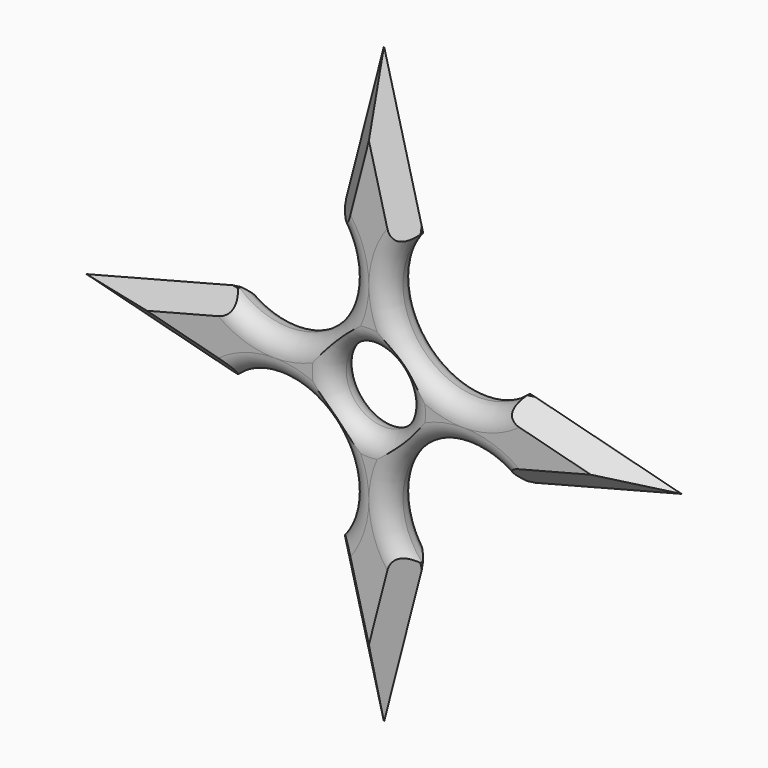
from build123d import *

# Parameters (mm, degrees)
F0_W         = 19.05
F0_H         = 25.4
F0_W_2       = 25.4
F0_H_2       = 19.05
F1_DEPTH     = 12.7
F3_D         = 50.8
F4_SIZE2     = 6.34999
F4_SIZE      = 6.34999
F5_T6_ANGLE  = 208.6059171241
F5_T8_ANGLE  = 208.6059171241
F5_T10_ANGLE = 208.6059171241
F5_T12_ANGLE = 208.6059171241
F5_T14_ANGLE = 208.6059171241
F5_T16_ANGLE = 208.6059171241
F5_T18_ANGLE = 208.6059171241
F5_T20_ANGLE = 208.6059171241


# Not quite as in the source:
# - a fillet or chamfer that OpenCascade refuses, or shapes differently, is made with other operations: its cross-section is extruded or revolved along the edge and cut away or added
# - a fillet or chamfer is up to 0.001 mm smaller than in the source, because OpenCascade refuses the exact size


with BuildPart() as f1:
    # F0 (on Front) → F1 (new body)
    with BuildSketch(Plane.XZ):
        with BuildLine():
            Line((-12.7, 12.7), (-4.87e-08, 12.7))
            Line((-4.87e-08, 12.7), (12.7, 12.7))
            Line((12.7, 12.7), (12.7, 14.1990316571))
            ThreePointArc((12.7, 14.1990316571), (0, 19.05), (-12.7, 14.1990316571))
            Line((-12.7, 14.1990316571), (-12.7, 12.7))
        make_face()
        with BuildLine():
            Line((-12.7, -12.7), (-12.7, 0))
            Line((-12.7, 0), (-12.7, 12.7))
            Line((-12.7, 12.7), (-14.1990316571, 12.7))
            ThreePointArc((-14.1990316571, 12.7), (-19.05, 0), (-14.1990316571, -12.7))
            Line((-14.1990316571, -12.7), (-12.7, -12.7))
        make_face()
        with BuildLine():
            Line((12.7, -12.7), (6e-10, -12.7))
            Line((6e-10, -12.7), (-12.7, -12.7))
            Line((-12.7, -12.7), (-12.7, -14.1990316571))
            ThreePointArc((-12.7, -14.1990316571), (0, -19.05), (12.7, -14.1990316571))
            Line((12.7, -14.1990316571), (12.7, -12.7))
        make_face()
        with BuildLine():
            Line((12.7, 12.7), (12.7, 0))
            Line((12.7, 0), (12.7, -12.7))
            Line((12.7, -12.7), (14.1990316571, -12.7))
            ThreePointArc((14.1990316571, -12.7), (17.7959834382, -6.7974608102), (19.05, 0))
            ThreePointArc((19.05, 0), (17.7959834382, 6.7974608102), (14.1990316571, 12.7))
            Line((14.1990316571, 12.7), (12.7, 12.7))
        make_face()
        with BuildLine():
            Line((12.7, -12.7), (12.7, 0))
            ThreePointArc((12.7, 0), (8.9802561213, -8.9802561208), (6e-10, -12.7))
            Line((6e-10, -12.7), (12.7, -12.7))
        make_face()
        with BuildLine():
            Line((-12.7, -12.7), (6e-10, -12.7))
            ThreePointArc((6e-10, -12.7), (-8.9802561208, -8.9802561213), (-12.7, 0))
            Line((-12.7, 0), (-12.7, -12.7))
        make_face()
        with BuildLine():
            ThreePointArc((-12.7, 0), (-8.9802561383, 8.9802561039), (-4.87e-08, 12.7))
            Line((-4.87e-08, 12.7), (-12.7, 12.7))
            Line((-12.7, 12.7), (-12.7, 0))
        make_face()
        with BuildLine():
            ThreePointArc((-4.87e-08, 12.7), (8.9802561039, 8.9802561383), (12.7, 0))
            Line((12.7, 0), (12.7, 12.7))
            Line((12.7, 12.7), (-4.87e-08, 12.7))
        make_face()
        with BuildLine():
            Line((12.7, 31.75), (12.7, 14.1990316571))
            ThreePointArc((12.7, 14.1990316571), (13.4703841816, 13.4703841816), (14.1990316571, 12.7))
            Line((14.1990316571, 12.7), (31.75, 12.7))
            Line((31.75, 12.7), (31.75, 31.75))
            Line((31.75, 31.75), (12.7, 31.75))
        make_face()
        with BuildLine():
            ThreePointArc((-12.7, 14.1990316571), (0, 19.05), (12.7, 14.1990316571))
            Line((12.7, 14.1990316571), (12.7, 31.75))
            Line((12.7, 31.75), (-12.7, 31.75))
            Line((-12.7, 31.75), (-12.7, 14.1990316571))
        make_face()
        with BuildLine():
            ThreePointArc((-14.1990316571, 12.7), (-13.4703841816, 13.4703841816), (-12.7, 14.1990316571))
            Line((-12.7, 14.1990316571), (-12.7, 31.75))
            Line((-12.7, 31.75), (-31.75, 31.75))
            Line((-31.75, 31.75), (-31.75, 12.7))
            Line((-31.75, 12.7), (-14.1990316571, 12.7))
        make_face()
        with BuildLine():
            ThreePointArc((-14.1990316571, -12.7), (-19.05, 0), (-14.1990316571, 12.7))
            Line((-14.1990316571, 12.7), (-31.75, 12.7))
            Line((-31.75, 12.7), (-31.75, -12.7))
            Line((-31.75, -12.7), (-14.1990316571, -12.7))
        make_face()
        with BuildLine():
            Line((-12.7, -31.75), (-12.7, -14.1990316571))
            ThreePointArc((-12.7, -14.1990316571), (-13.4703841816, -13.4703841816), (-14.1990316571, -12.7))
            Line((-14.1990316571, -12.7), (-31.75, -12.7))
            Line((-31.75, -12.7), (-31.75, -31.75))
            Line((-31.75, -31.75), (-12.7, -31.75))
        make_face()
        with BuildLine():
            Line((12.7, -31.75), (12.7, -14.1990316571))
            ThreePointArc((12.7, -14.1990316571), (0, -19.05), (-12.7, -14.1990316571))
            Line((-12.7, -14.1990316571), (-12.7, -31.75))
            Line((-12.7, -31.75), (12.7, -31.75))
        make_face()
        with BuildLine():
            ThreePointArc((14.1990316571, -12.7), (13.4703841816, -13.4703841816), (12.7, -14.1990316571))
            Line((12.7, -14.1990316571), (12.7, -31.75))
            Line((12.7, -31.75), (31.75, -31.75))
            Line((31.75, -31.75), (31.75, -12.7))
            Line((31.75, -12.7), (14.1990316571, -12.7))
        make_face()
        with BuildLine():
            ThreePointArc((19.05, 0), (17.7959834382, -6.7974608102), (14.1990316571, -12.7))
            Line((14.1990316571, -12.7), (31.75, -12.7))
            Line((31.75, -12.7), (31.75, 12.7))
            Line((31.75, 12.7), (14.1990316571, 12.7))
            ThreePointArc((14.1990316571, 12.7), (17.7959834382, 6.7974608102), (19.05, 0))
        make_face()
        with Locations((41.275, 0)):
            Rectangle(F0_W, F0_H)
        Polygon((50.8, 12.7), (50.8, -12.7), (99.9868884968, 0), align=None)
        Polygon((-12.7, 50.8), (12.7, 50.8), (0, 99.9868884968), align=None)
        with Locations((0, 41.275)):
            Rectangle(F0_W_2, F0_H_2)
        with Locations((-41.275, 0)):
            Rectangle(F0_W, F0_H)
        Polygon((-50.8, -12.7), (-50.8, 12.7), (-99.9868884968, 0), align=None)
        Polygon((0, -99.9868884968), (12.7, -50.8), (-12.7, -50.8), align=None)
        with Locations((0, -41.275)):
            Rectangle(F0_W_2, F0_H_2)
        with BuildLine():
            Line((14.1990316571, -12.7), (12.7, -12.7))
            Line((12.7, -12.7), (12.7, -14.1990316571))
            ThreePointArc((12.7, -14.1990316571), (13.4703841816, -13.4703841816), (14.1990316571, -12.7))
        make_face()
        with BuildLine():
            Line((-12.7, -14.1990316571), (-12.7, -12.7))
            Line((-12.7, -12.7), (-14.1990316571, -12.7))
            ThreePointArc((-14.1990316571, -12.7), (-13.4703841816, -13.4703841816), (-12.7, -14.1990316571))
        make_face()
        with BuildLine():
            Line((-14.1990316571, 12.7), (-12.7, 12.7))
            Line((-12.7, 12.7), (-12.7, 14.1990316571))
            ThreePointArc((-12.7, 14.1990316571), (-13.4703841816, 13.4703841816), (-14.1990316571, 12.7))
        make_face()
        with BuildLine():
            Line((12.7, 14.1990316571), (12.7, 12.7))
            Line((12.7, 12.7), (14.1990316571, 12.7))
            ThreePointArc((14.1990316571, 12.7), (13.4703841816, 13.4703841816), (12.7, 14.1990316571))
        make_face()
    extrude(amount=F1_DEPTH)

    # F3 (through all)
    with Locations(Plane.XZ.offset(12.7)):
        with Locations((-31.75, 31.75), (-31.75, -31.75), (31.75, -31.75), (31.75, 31.75)):
            Hole(F3_D / 2)

    # F4 (size 6.35 and 6.35 in the source; OpenCascade refuses exactly that, so slightly less here)
    f4_edges = [f1.edges().sort_by_distance(p)[0] for p in [
        (-75.393444, -12.7, 6.35),
        (-75.393444, -12.7, -6.35),
        (-75.393444, 0, -6.35),
        (-75.393444, 0, 6.35),
        (6.35, -12.7, 75.393444),
        (-6.35, -12.7, 75.393444),
        (-6.35, 0, 75.393444),
        (6.35, 0, 75.393444),
        (75.393444, 0, 6.35),
        (75.393444, -12.7, 6.35),
        (75.393444, 0, -6.35),
        (75.393444, -12.7, -6.35),
        (-6.35, 0, -75.393444),
        (6.35, 0, -75.393444),
        (6.35, -12.7, -75.393444),
        (-6.35, -12.7, -75.393444),
    ]]
    chamfer(f4_edges, length=F4_SIZE, length2=F4_SIZE2)

    # F5: fillet of radius 6.35 on 10 edges, made by hand

    # F5_s1 → F5_t2 (revolve, cut)
    with BuildSketch(Plane.YZ):
        with BuildLine():
            ThreePointArc((-6.35, 12.7), (-1.8598719395, 14.5598719395), (0, 19.05))
            Line((0, 19.05), (0, 12.7))
            Line((0, 12.7), (-6.35, 12.7))
        make_face()
    revolve(axis=Axis((0, 0, 0), (0, 1, 0)), mode=Mode.SUBTRACT)

    # F5_s3 → F5_t4 (revolve, cut)
    with BuildSketch(Plane.YZ):
        with BuildLine():
            ThreePointArc((-12.7, 19.05), (-10.8401280605, 14.5598719395), (-6.35, 12.7))
            Line((-6.35, 12.7), (-12.7, 12.7))
            Line((-12.7, 12.7), (-12.7, 19.05))
        make_face()
    revolve(axis=Axis((0, -12.7, 0), (0, 1, 0)), mode=Mode.SUBTRACT)

    # F5_s5 → F5_t6 (revolve, cut)
    with BuildSketch(Plane(origin=(-37.4128674881, 0, 22.2115222373), x_dir=(0, 1, 0), z_dir=(-0.8598786332, 0, 0.5104985173))):
        with BuildLine():
            ThreePointArc((-12.7, -42.8428186777), (-10.8401280605, -38.3526906172), (-6.35, -36.4928186777))
            Line((-6.35, -36.4928186777), (-12.7, -36.4928186777))
            Line((-12.7, -36.4928186777), (-12.7, -42.8428186777))
        make_face()
    revolve(axis=Axis((-31.75, -12.7, 31.75), (0, 1, 0)), revolution_arc=F5_T6_ANGLE, mode=Mode.SUBTRACT)

    # F5_s7 → F5_t8 (revolve, cut)
    with BuildSketch(Plane(origin=(37.4128674881, 0, 22.2115222373), x_dir=(0, 1, 0), z_dir=(0.8598786332, 0, 0.5104985173))):
        with BuildLine():
            ThreePointArc((-12.7, 42.8428186777), (-10.8401280605, 38.3526906172), (-6.35, 36.4928186777))
            Line((-6.35, 36.4928186777), (-12.7, 36.4928186777))
            Line((-12.7, 36.4928186777), (-12.7, 42.8428186777))
        make_face()
    revolve(axis=Axis((31.75, -12.7, 31.75), (0, -1, 0)), revolution_arc=F5_T8_ANGLE, mode=Mode.SUBTRACT)

    # F5_s9 → F5_t10 (revolve, cut)
    with BuildSketch(Plane(origin=(-22.2115222373, 0, -37.4128674881), x_dir=(0, 1, 0), z_dir=(-0.5104985173, 0, -0.8598786332))):
        with BuildLine():
            ThreePointArc((-12.7, -42.8428186777), (-10.8401280605, -38.3526906172), (-6.35, -36.4928186777))
            Line((-6.35, -36.4928186777), (-12.7, -36.4928186777))
            Line((-12.7, -36.4928186777), (-12.7, -42.8428186777))
        make_face()
    revolve(axis=Axis((-31.75, -12.7, -31.75), (0, 1, 0)), revolution_arc=F5_T10_ANGLE, mode=Mode.SUBTRACT)

    # F5_s11 → F5_t12 (revolve, cut)
    with BuildSketch(Plane(origin=(22.2115222373, 0, -37.4128674881), x_dir=(0, 1, 0), z_dir=(0.5104985173, 0, -0.8598786332))):
        with BuildLine():
            ThreePointArc((-12.7, 42.8428186777), (-10.8401280605, 38.3526906172), (-6.35, 36.4928186777))
            Line((-6.35, 36.4928186777), (-12.7, 36.4928186777))
            Line((-12.7, 36.4928186777), (-12.7, 42.8428186777))
        make_face()
    revolve(axis=Axis((31.75, -12.7, -31.75), (0, -1, 0)), revolution_arc=F5_T12_ANGLE, mode=Mode.SUBTRACT)

    # F5_s13 → F5_t14 (revolve, cut)
    with BuildSketch(Plane(origin=(-22.2115222373, 0, 37.4128674881), x_dir=(0, 1, 0), z_dir=(-0.5104985173, 0, 0.8598786332))):
        with BuildLine():
            ThreePointArc((-6.35, 36.4928186777), (-1.8598719395, 38.3526906172), (0, 42.8428186777))
            Line((0, 42.8428186777), (0, 36.4928186777))
            Line((0, 36.4928186777), (-6.35, 36.4928186777))
        make_face()
    revolve(axis=Axis((-31.75, 0, 31.75), (0, -1, 0)), revolution_arc=F5_T14_ANGLE, mode=Mode.SUBTRACT)

    # F5_s15 → F5_t16 (revolve, cut)
    with BuildSketch(Plane(origin=(37.4128674881, 0, 22.2115222373), x_dir=(0, 1, 0), z_dir=(0.8598786332, 0, 0.5104985173))):
        with BuildLine():
            ThreePointArc((-6.35, 36.4928186777), (-1.8598719395, 38.3526906172), (0, 42.8428186777))
            Line((0, 42.8428186777), (0, 36.4928186777))
            Line((0, 36.4928186777), (-6.35, 36.4928186777))
        make_face()
    revolve(axis=Axis((31.75, 0, 31.75), (0, -1, 0)), revolution_arc=F5_T16_ANGLE, mode=Mode.SUBTRACT)

    # F5_s17 → F5_t18 (revolve, cut)
    with BuildSketch(Plane(origin=(-37.4128674881, 0, -22.2115222373), x_dir=(0, 1, 0), z_dir=(-0.8598786332, 0, -0.5104985173))):
        with BuildLine():
            ThreePointArc((-6.35, 36.4928186777), (-1.8598719395, 38.3526906172), (0, 42.8428186777))
            Line((0, 42.8428186777), (0, 36.4928186777))
            Line((0, 36.4928186777), (-6.35, 36.4928186777))
        make_face()
    revolve(axis=Axis((-31.75, 0, -31.75), (0, -1, 0)), revolution_arc=F5_T18_ANGLE, mode=Mode.SUBTRACT)

    # F5_s19 → F5_t20 (revolve, cut)
    with BuildSketch(Plane(origin=(22.2115222373, 0, -37.4128674881), x_dir=(0, 1, 0), z_dir=(0.5104985173, 0, -0.8598786332))):
        with BuildLine():
            ThreePointArc((-6.35, 36.4928186777), (-1.8598719395, 38.3526906172), (0, 42.8428186777))
            Line((0, 42.8428186777), (0, 36.4928186777))
            Line((0, 36.4928186777), (-6.35, 36.4928186777))
        make_face()
    revolve(axis=Axis((31.75, 0, -31.75), (0, -1, 0)), revolution_arc=F5_T20_ANGLE, mode=Mode.SUBTRACT)


solid = f1.part
